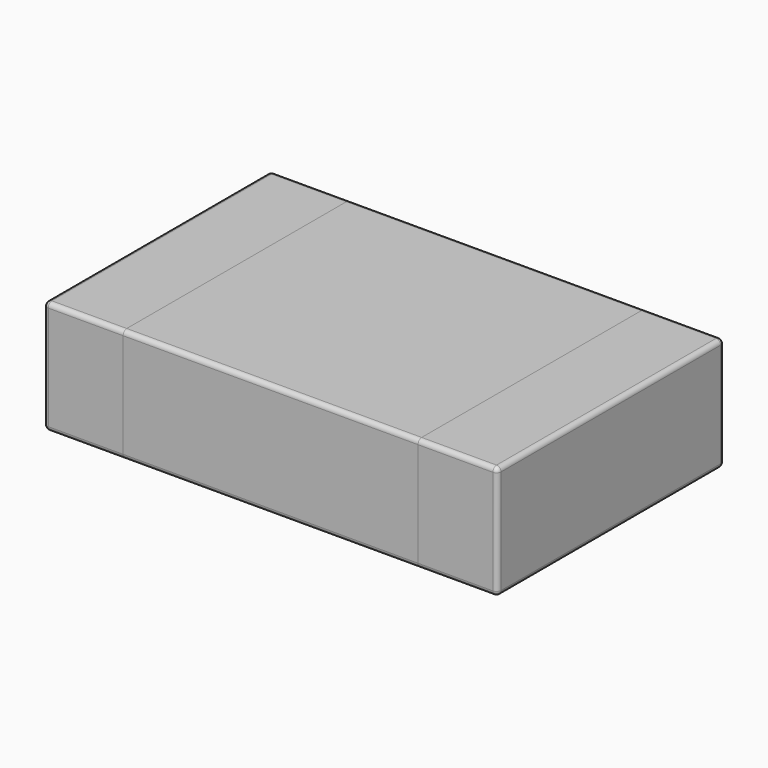
from build123d import *

# Parameters (mm, degrees)
F2_W     = 1.3
F2_H     = 1.25
F3_DEPTH = 0.48
F2_W_2   = 0.35
F4_DEPTH = 0.5
F5_DEPTH = 0.5
F6_DEPTH = 0.02
F7_R     = 0.01999
F7_2_R   = 0.01999
F7_3_R   = 0.01999
F7_4_R   = 0.01999


# Not quite as in the source:
# - a fillet or chamfer is up to 0.001 mm smaller than in the source, because OpenCascade refuses the exact size


with BuildPart() as f3:
    # F2 (on Top) → F3 (new body)
    with BuildSketch(Plane.XY):
        Rectangle(F2_W, F2_H)
    extrude(amount=F3_DEPTH)


with BuildPart() as f4:
    # F2 (on Top) → F4 (new body)
    with BuildSketch(Plane.XY):
        with Locations((-0.825, 0)):
            Rectangle(F2_W_2, F2_H)
    extrude(amount=F4_DEPTH)

    # F7 (radius 0.02 in the source; OpenCascade refuses exactly that, so slightly less here)
    f7_edges = [f4.edges().sort_by_distance(p)[0] for p in [
        (-0.825, -0.625, 0.5),
        (-1, 0.625, 0.25),
        (-1, -0.625, 0.25),
        (-1, 0, 0),
        (-1, 0, 0.5),
        (-0.825, 0.625, 0.5),
        (-0.825, 0.625, 0),
        (-0.825, -0.625, 0),
    ]]
    fillet(f7_edges, radius=F7_R)


with BuildPart() as f5:
    # F2 (on Top) → F5 (new body)
    with BuildSketch(Plane.XY):
        with Locations((0.825, 0)):
            Rectangle(F2_W_2, F2_H)
    extrude(amount=F5_DEPTH)

    # F7#2 (radius 0.02 in the source; OpenCascade refuses exactly that, so slightly less here)
    f7_2_edges = [f5.edges().sort_by_distance(p)[0] for p in [
        (0.825, -0.625, 0.5),
        (1, -0.625, 0.25),
        (1, 0.625, 0.25),
        (1, 0, 0),
        (1, 0, 0.5),
        (0.825, 0.625, 0.5),
        (0.825, 0.625, 0),
        (0.825, -0.625, 0),
    ]]
    fillet(f7_2_edges, radius=F7_2_R)


with BuildPart() as f6:
    # F6 (new): a face of the model
    f6_faces = [f3.part.faces().sort_by_distance(p)[0] for p in [
        (0, 0, 0.48),
    ]]
    extrude(f6_faces, amount=F6_DEPTH)

    # F7#4 (radius 0.02 in the source; OpenCascade refuses exactly that, so slightly less here)
    f7_4_edges = [f6.edges().sort_by_distance(p)[0] for p in [
        (0, -0.625, 0.5),
        (0, 0.625, 0.5),
    ]]
    fillet(f7_4_edges, radius=F7_4_R)


with BuildPart() as f3_1:
    add(f3.part)

    # F7#3 (radius 0.02 in the source; OpenCascade refuses exactly that, so slightly less here)
    f7_3_edges = [f3_1.edges().sort_by_distance(p)[0] for p in [
        (0, 0.625, 0),
        (0, -0.625, 0),
    ]]
    fillet(f7_3_edges, radius=F7_3_R)


solid = Compound([f4.part, f5.part, f6.part, f3_1.part])
